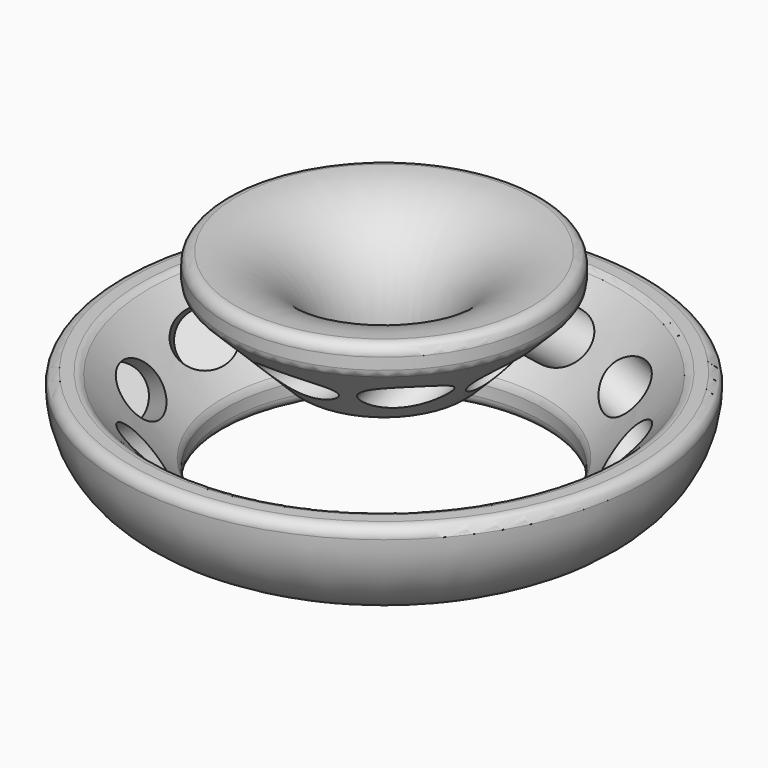
from build123d import *

# Parameters (mm, degrees)
F0_R             = 63.5
F0_R_2           = 38.1
F1_DEPTH         = 25.4
F2_SIZE          = 19.05
F5_R             = 6.35
F6_DEPTH         = 17.78
F6_COPIES_COUNT  = 12
F8_R             = 38.1
F8_R_2           = 12.7
F9_DEPTH         = 25.4
F10_SIZE         = 19.05
F11_R            = 22.86
F12_R            = 2.53999
F13_R            = 22.86
F14_R            = 2.53999
F17_R            = 6.35
F18_DEPTH        = 11.43
F18_DEPTH_BACK   = 79.8263822203
F18_COPIES_COUNT = 8
F19_DEPTH        = 12.7


# Not quite as in the source:
# - a fillet or chamfer is up to 0.001 mm smaller than in the source, because OpenCascade refuses the exact size
# - a pattern or mirror of a feature is missing from the dataset's text; its kind, count and spacing are read off the source's solid


with BuildPart() as f1:
    # F0 (on Top) → F1 (new body)
    with BuildSketch(Plane.XY):
        Circle(F0_R)
        Circle(F0_R_2, mode=Mode.SUBTRACT)
    extrude(amount=F1_DEPTH)

    # F2
    f2_edges = [f1.edges().sort_by_distance(p)[0] for p in [
        (-38.1, 0, 25.4),
    ]]
    chamfer(f2_edges, length=F2_SIZE)

    # F5 (on face) → F6 (cut)
    with BuildSketch(Plane(origin=(8.846285122, 6.2552681981, -6.2552681981), x_dir=(-0.4082482905, 0.8660254038, 0.2886751346), z_dir=(0.7071067812, 0.5, -0.5))):
        with Locations((43.1141834706, 15.3094567358)):
            Circle(F5_R)
    f6 = extrude(amount=F6_DEPTH, mode=Mode.SUBTRACT)

    # F6_copies: F6 ×12 about axis
    f6_copies_axis = Axis((0, 0, 0), (0, 0, 1))
    for i in range(1, F6_COPIES_COUNT):
        add(f6.rotate(f6_copies_axis, i * 360 / F6_COPIES_COUNT), mode=Mode.SUBTRACT)

    # F11
    f11_edges = [f1.edges().sort_by_distance(p)[0] for p in [
        (-63.5, 0, 0),
    ]]
    fillet(f11_edges, radius=F11_R)

    # F12 (radius 2.54 in the source; OpenCascade refuses exactly that, so slightly less here)
    f12_edges = [f1.edges().sort_by_distance(p)[0] for p in [
        (-63.5, 0, 25.4),
        (-57.15, 0, 25.4),
        (-38.1, 0, 6.35),
        (-38.1, 0, 0),
    ]]
    fillet(f12_edges, radius=F12_R)


with BuildPart() as f9:
    # F8 (on face) → F9 (new body)
    with BuildSketch(Plane.XY.offset(25.4)):
        Circle(F8_R)
        Circle(F8_R_2, mode=Mode.SUBTRACT)
    extrude(amount=F9_DEPTH)

    # F10
    f10_edges = [f9.edges().sort_by_distance(p)[0] for p in [
        (-38.1, 0, 25.4),
    ]]
    chamfer(f10_edges, length=F10_SIZE)

    # F13
    f13_edges = [f9.edges().sort_by_distance(p)[0] for p in [
        (-12.7, 0, 50.8),
    ]]
    fillet(f13_edges, radius=F13_R)

    # F14 (radius 2.54 in the source; OpenCascade refuses exactly that, so slightly less here)
    f14_edges = [f9.edges().sort_by_distance(p)[0] for p in [
        (-38.1, 0, 44.45),
        (-19.05, 0, 25.4),
        (-12.7, 0, 25.4),
        (-38.1, 0, 50.8),
    ]]
    fillet(f14_edges, radius=F14_R)

    # F17 (on face) → F18 (cut, two sides)
    with BuildSketch(Plane(origin=(-2.2444287761, -1.5870508075, 1.5870508075), x_dir=(-0.4082482905, 0.8660254038, 0.2886751346), z_dir=(0.7071067812, 0.5, -0.5))) as f18_sk:
        with Locations((34.2830551374, 28.1292454416)):
            Circle(F17_R)
    f18 = extrude(amount=-F18_DEPTH, mode=Mode.SUBTRACT) + extrude(f18_sk.sketch, amount=F18_DEPTH_BACK, mode=Mode.SUBTRACT)

    # F18_copies: F18 ×8 about axis
    f18_copies_axis = Axis((0, 0, 0), (0, 0, 1))
    for i in range(1, F18_COPIES_COUNT):
        add(f18.rotate(f18_copies_axis, i * 360 / F18_COPIES_COUNT), mode=Mode.SUBTRACT)


with BuildPart() as f19:
    # F5 (on face) → F19 (new body)
    with BuildSketch(Plane(origin=(8.846285122, 6.2552681981, -6.2552681981), x_dir=(-0.4082482905, 0.8660254038, 0.2886751346), z_dir=(0.7071067812, 0.5, -0.5))):
        with Locations((43.1141834706, 15.3094567358)):
            Circle(F5_R)
    extrude(amount=F19_DEPTH)


solid = Compound([f1.part, f9.part, f19.part])
